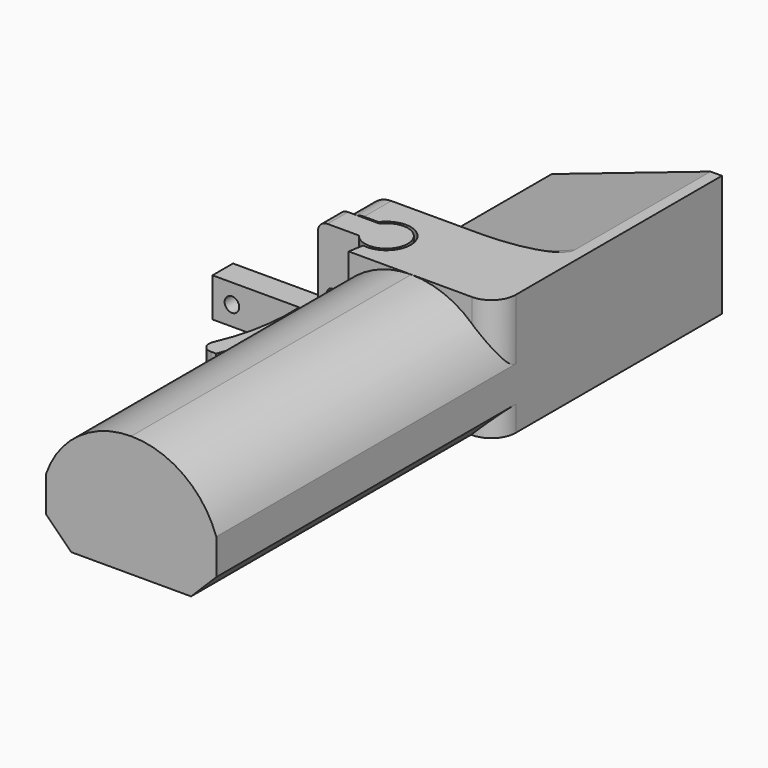
from build123d import *

# Parameters (mm, degrees)
F0_W         = 35
F0_H         = 100
F1_DEPTH     = 25
F3_DEPTH     = 40
F5_DEPTH     = 25.001
F6_W         = 6
F6_H         = 25
F6_R         = 1.5
F7_DEPTH     = 7
F9_DEPTH     = 25
F10_R        = 1.0999994278
F11_DEPTH    = 52.641
F13_DEPTH    = 8
F14_T1_DEPTH = 5.28
F14_T3_DEPTH = 24.0296074828
F14_T5_DEPTH = 15.28
F15_DEPTH    = 30
F17_DEPTH    = 72
F18_R        = 5
F19_R        = 1.5
F20_DEPTH    = 82.6410001


# Not quite as in the source:
# - a fillet or chamfer that OpenCascade refuses, or shapes differently, is made with other operations: its cross-section is extruded or revolved along the edge and cut away or added


with BuildPart() as f1:
    # F0 (on Top) → F1 (new body)
    with BuildSketch(Plane.XY):
        Rectangle(F0_W, F0_H)
    extrude(amount=F1_DEPTH)

    # F2 (on face) → F3 (cut)
    with BuildSketch(Plane(origin=(0, 50, 0), x_dir=(-1, 0, 0), z_dir=(0, 1, 0))):
        Polygon((15.5, 12.5), (-15.5, 23), (-15.5, 2), align=None)
        Polygon((17.5, 25), (-15.1704846289, 25), (17.5, 13.9341906902), align=None)
    extrude(amount=-F3_DEPTH, mode=Mode.SUBTRACT)

    # F4 (on face) → F5 (cut, through all)
    with BuildSketch(Plane.XY.offset(25)):
        with BuildLine():
            ThreePointArc((-12.3448190756, -4.9281112741), (-8.2769653568, -3.822570822), (-6.5, 0))
            ThreePointArc((-6.5, 0), (-9.9188611699, 4.7434164903), (-15.5, 3))
            Line((-15.5, 3), (-15.5, -3))
            ThreePointArc((-15.5, -3), (-14.1071960494, -4.2664421665), (-12.3448190756, -4.9281112741))
        make_face()
        with BuildLine():
            Line((-15.5, -3), (-15.5, 3))
            ThreePointArc((-15.5, 3), (-16.5, 0), (-15.5, -3))
        make_face()
        with BuildLine():
            ThreePointArc((-15.5, -3), (-16.5, 0), (-15.5, 3))
            Line((-15.5, 3), (-19.5, 3))
            Line((-19.5, 3), (-19.5, -3))
            Line((-19.5, -3), (-17.5, -3))
            Line((-17.5, -3), (-15.5, -3))
        make_face()
        with BuildLine():
            Line((-17.5, -35), (-12.3448190756, -4.9281112741))
            ThreePointArc((-12.3448190756, -4.9281112741), (-14.1071960494, -4.2664421665), (-15.5, -3))
            Line((-15.5, -3), (-17.5, -3))
            Line((-17.5, -3), (-17.5, -35))
        make_face()
    extrude(amount=-F5_DEPTH, mode=Mode.SUBTRACT)

    # F6 (on face) → F7 (join, through all)
    with BuildSketch(Plane.XZ.offset(-3)):
        with Locations((-20.5, 12.5)):
            Rectangle(F6_W, F6_H)
        with Locations((-20.5, 12.5)):
            Circle(F6_R, mode=Mode.SUBTRACT)
    extrude(amount=-F7_DEPTH)

    # F15 (add): a face of the model
    f15_faces = [f1.faces().sort_by_distance(p)[0] for p in [
        (0, -50, 12.5),
    ]]
    extrude(f15_faces, amount=F15_DEPTH)

    # F16 (on face) → F17 (cut)
    with BuildSketch(Plane.XZ.offset(80)):
        with BuildLine():
            ThreePointArc((0, 25), (10.7529065838, 21.5540692173), (17.5, 12.5))
            Line((17.5, 12.5), (17.5, 25))
            Line((17.5, 25), (0, 25))
        make_face()
        with BuildLine():
            ThreePointArc((-17.5, 12.5), (-10.7529065838, 21.5540692173), (0, 25))
            Line((0, 25), (-17.5, 25))
            Line((-17.5, 25), (-17.5, 12.5))
        make_face()
        Polygon((-12.3223304703, 0), (-17.5, 5.1776695297), (-17.5, 0), align=None)
        Polygon((17.5, 0), (17.5, 5.1776695297), (12.3223304703, 0), align=None)
    extrude(amount=-F17_DEPTH, mode=Mode.SUBTRACT)

    # F18
    f18_edges = [f1.edges().sort_by_distance(p)[0] for p in [
        (17.5, -8, 18.75),
        (17.5, -8, 2.588835),
        (-1.164758, 10, 19.467095),
        (-23.5, 6.5, 0),
        (-23.5, 6.5, 25),
    ]]
    fillet(f18_edges, radius=F18_R)


with BuildPart() as f9:
    # F8 (on Top) → F9 (new body, through all)
    with BuildSketch(Plane.XY):
        with BuildLine():
            Line((-23.5, -2.64), (-15.02, -2.64))
            ThreePointArc((-15.02, -2.64), (-7.1, 0), (-15.02, 2.64))
            Line((-15.02, 2.64), (-23.5, 2.64))
            Line((-23.5, 2.64), (-23.5, -2.64))
        make_face()
    extrude(amount=F9_DEPTH)

    # F10 (on face) → F11 (cut, through all)
    with BuildSketch(Plane(origin=(0, 2.64, 0), x_dir=(-1, 0, 0), z_dir=(0, 1, 0))):
        with Locations((20.5, 12.5)):
            Circle(F10_R)
    extrude(amount=-F11_DEPTH, mode=Mode.SUBTRACT)

    # F12 (on face) → F13 (join)
    with BuildSketch(Plane(origin=(0, 0, 0), x_dir=(1, 0, 0), z_dir=(0, 0, -1))):
        with BuildLine():
            ThreePointArc((-23.5, 2.64), (-24.5610181297, 13.3015957041), (-27.7024523358, 23.5449727625))
            Line((-27.7024523358, 23.5449727625), (-31.957603991, 23.5449727625))
            ThreePointArc((-31.957603991, 23.5449727625), (-28.1854810092, 13.4160571698), (-27.3485612124, 2.64))
            Line((-27.3485612124, 2.64), (-45.1639331877, 2.64))
            Line((-45.1639331877, 2.64), (-45.1639331877, -2.64))
            Line((-45.1639331877, -2.64), (-23.5, -2.64))
            Line((-23.5, -2.64), (-23.5, 2.64))
        make_face()
    extrude(amount=-F13_DEPTH)

    # F14: fillet of radius 2 on 3 edges, made by hand

    # F14_s2 → F14_t1 (join)
    with BuildSketch(Plane.XZ.offset(-2.64)):
        with BuildLine():
            ThreePointArc((-25.5, 8), (-24.0857864376, 8.5857864376), (-23.5, 10))
            Line((-23.5, 10), (-23.5, 8))
            Line((-23.5, 8), (-25.5, 8))
        make_face()
    extrude(amount=F14_T1_DEPTH)

    # F14_s4 → F14_t3 (cut)
    with BuildSketch(Plane.XY.offset(-8.0148037414)):
        with BuildLine():
            ThreePointArc((-28.7516824945, -23.5449727625), (-30.4271988015, -22.6370556829), (-30.5814852362, -20.7376178675))
            ThreePointArc((-30.5814852362, -20.7376178675), (-31.2413053207, -22.1551377475), (-31.957603991, -23.5449727625))
            Line((-31.957603991, -23.5449727625), (-28.7516824945, -23.5449727625))
        make_face()
    extrude(amount=F14_T3_DEPTH, mode=Mode.SUBTRACT)

    # F14_s6 → F14_t5 (cut)
    with BuildSketch(Plane.XZ.offset(-7.64)):
        with BuildLine():
            ThreePointArc((-21.5, 25), (-22.9142135624, 24.4142135624), (-23.5, 23))
            Line((-23.5, 23), (-23.5, 25))
            Line((-23.5, 25), (-21.5, 25))
        make_face()
    extrude(amount=F14_T5_DEPTH, mode=Mode.SUBTRACT)

    # F19 (on face) → F20 (cut, through all)
    with BuildSketch(Plane(origin=(0, 2.64, 0), x_dir=(-1, 0, 0), z_dir=(0, 1, 0))):
        with Locations((41.1639331877, 4)):
            Circle(F19_R)
    extrude(amount=-F20_DEPTH, mode=Mode.SUBTRACT)


solid = Compound([f1.part, f9.part])
